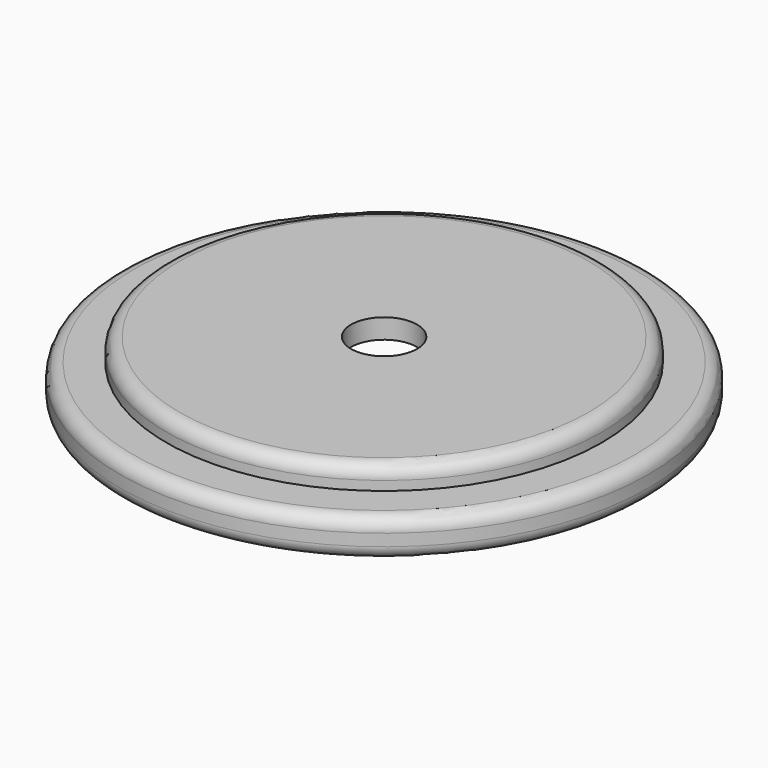
from build123d import *

# Parameters (mm, degrees)
F2_R     = 1
F3_R     = 2.5
F4_DEPTH = 1.501


# Not quite as in the source:
# - a feature names something its author has since deleted; it is built from what else it names


with BuildPart() as f1:
    # F0 (on Front) → F1 (revolve)
    with BuildSketch(Plane.XZ):
        Polygon((15.1, 3.1), (15.1, 0), (20, 0), (20, 2.9), (16.5, 2.9), (16.5, 4.6), (0, 4.6), (0, 3.1), align=None)
    revolve(axis=Axis((0, 0, 3.0650238041), (0, 0, -1)))

    # F2
    f2_edges = [f1.edges().sort_by_distance(p)[0] for p in [
        (-15.1, 0, 0),
        (-20, 0, 0),
        (-16.5, 0, 4.6),
        (-20, 0, 2.9),
    ]]
    fillet(f2_edges, radius=F2_R)

    # F3 (on face) → F4 (cut, through all)
    with BuildSketch(Plane(origin=(0, 0, 3.1), x_dir=(1, 0, 0), z_dir=(0, 0, -1))):
        Circle(F3_R)
    extrude(amount=-F4_DEPTH, mode=Mode.SUBTRACT)


solid = f1.part
